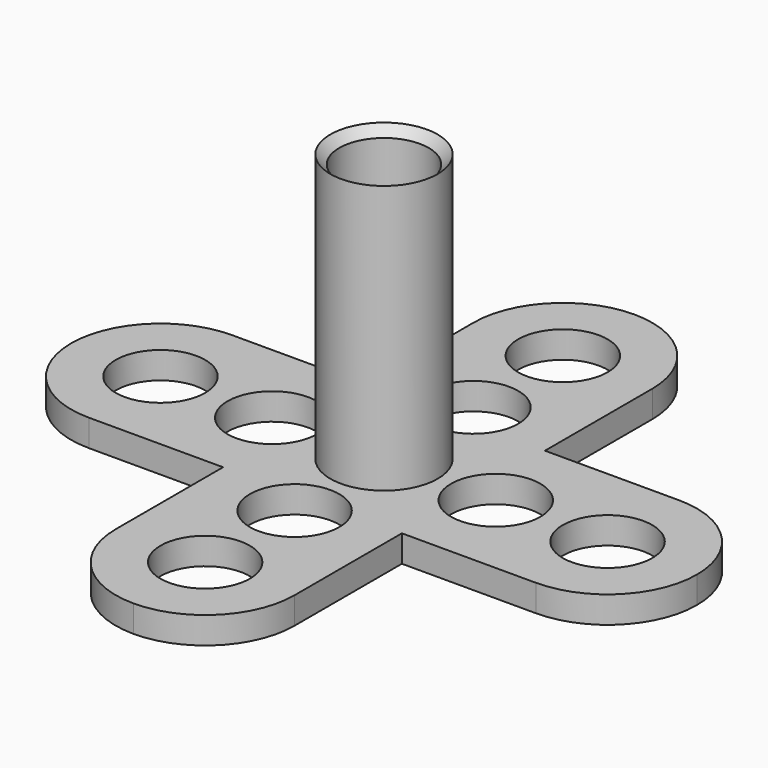
from build123d import *

# Parameters (mm, degrees)
F1_DEPTH = 3
F3_D     = 10
F4_R     = 6
F4_R_2   = 5
F5_DEPTH = 30
F6_SIZE  = 0.99999


# Not quite as in the source:
# - a fillet or chamfer is up to 0.001 mm smaller than in the source, because OpenCascade refuses the exact size


with BuildPart() as f1:
    # F0 (on Top) → F1 (new body)
    with BuildSketch(Plane.XY):
        with BuildLine():
            Line((10, 10), (10, 25))
            ThreePointArc((10, 25), (7.0710678119, 32.0710678119), (0, 35))
            ThreePointArc((0, 35), (-7.0710678119, 32.0710678119), (-10, 25))
            Line((-10, 25), (-10, 10))
            Line((-10, 10), (-25, 10))
            ThreePointArc((-25, 10), (-32.0710678119, 7.0710678119), (-35, 0))
            ThreePointArc((-35, 0), (-32.0710678119, -7.0710678119), (-25, -10))
            Line((-25, -10), (-10, -10))
            Line((-10, -10), (-10, -25))
            ThreePointArc((-10, -25), (-7.0710678119, -32.0710678119), (0, -35))
            ThreePointArc((0, -35), (7.0710678119, -32.0710678119), (10, -25))
            Line((10, -25), (10, -10))
            Line((10, -10), (25, -10))
            ThreePointArc((25, -10), (32.0710678119, -7.0710678119), (35, 0))
            ThreePointArc((35, 0), (32.0710678119, 7.0710678119), (25, 10))
            Line((25, 10), (10, 10))
        make_face()
    extrude(amount=F1_DEPTH)

    # F3 (through all)
    with Locations(Plane.XY.offset(3)):
        with Locations((-25, 0), (-12.5, 0), (0, 25), (0, 12.5), (12.5, 0), (25, 0), (0, -12.5), (0, -25)):
            Hole(F3_D / 2)

    # F4 (on face) → F5 (join)
    with BuildSketch(Plane.XY.offset(3)):
        Circle(F4_R)
        Circle(F4_R_2, mode=Mode.SUBTRACT)
    extrude(amount=F5_DEPTH)

    # F6 (size 1 in the source; OpenCascade refuses exactly that, so slightly less here)
    f6_edges = [f1.edges().sort_by_distance(p)[0] for p in [
        (-5, 0, 33),
    ]]
    chamfer(f6_edges, length=F6_SIZE)


solid = f1.part
